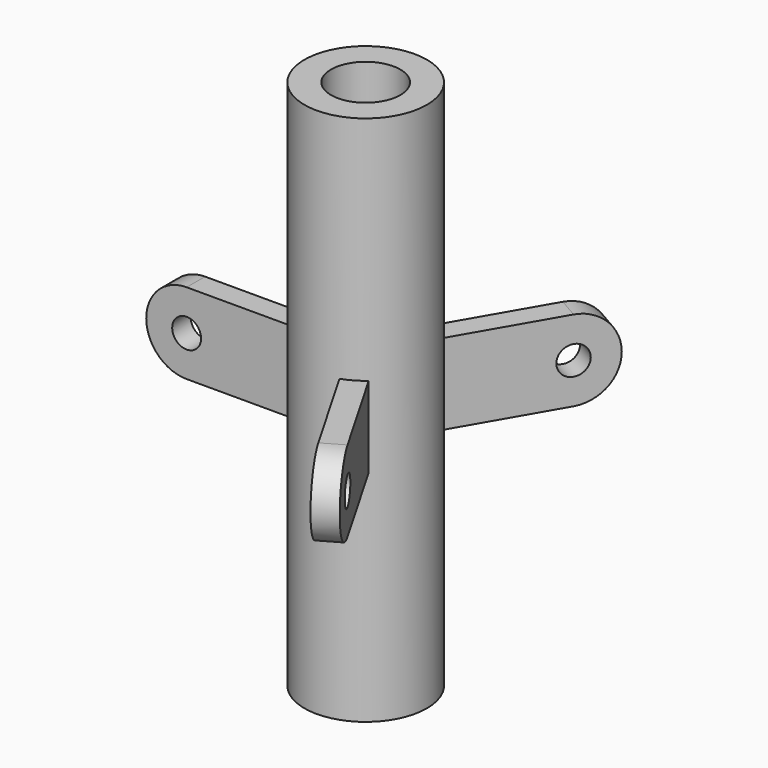
from build123d import *

# Parameters (mm, degrees)
F0_R            = 10.6
F1_DEPTH        = 92
F2_R            = 6
F3_DEPTH        = 98.1
F5_DEPTH        = 2
F5_COPIES_COUNT = 3
F7_R            = 2.5
F8_DEPTH        = 4
F9_R            = 2.5
F10_DEPTH       = 4
F11_R           = 2.5
F12_DEPTH       = 4


# Not quite as in the source:
# - a feature of the source that left no trace in its solid (it failed there, or was rolled back) is left out
# - a pattern or mirror of a feature is missing from the dataset's text; its kind, count and spacing are read off the source's solid


with BuildPart() as f1:
    # F0 (on Top) → F1 (new body)
    with BuildSketch(Plane.XY):
        Circle(F0_R)
    extrude(amount=F1_DEPTH)

    # F2 (on face) → F3 (cut)
    with BuildSketch(Plane(origin=(0, 0, 0), x_dir=(1, 0, 0), z_dir=(0, 0, -1))):
        Circle(F2_R)
    extrude(amount=-F3_DEPTH, mode=Mode.SUBTRACT)

    # F4 (on Front) → F5 (join, symmetric)
    with BuildSketch(Plane.XZ):
        with BuildLine():
            Line((-9.7803492099, 52), (-29.4, 52))
            ThreePointArc((-29.4, 52), (-36.4, 45), (-29.4, 38))
            Line((-29.4, 38), (-9.7803492099, 38))
            Line((-9.7803492099, 38), (-9.7803492099, 52))
        make_face()
    f5 = extrude(amount=F5_DEPTH, both=True)

    # F5_copies: F5 ×3 about axis
    f5_copies_axis = Axis((0, 0, 0), (0, 0, 1))
    for i in range(1, F5_COPIES_COUNT):
        add(f5.rotate(f5_copies_axis, i * 360 / F5_COPIES_COUNT))

    # F7 (on face) → F8 (cut, through all)
    with BuildSketch(Plane.XZ.offset(2)):
        with Locations((-29.4, 45)):
            Circle(F7_R)
    extrude(amount=-F8_DEPTH, mode=Mode.SUBTRACT)

    # F9 (on face) → F10 (cut, through all)
    with BuildSketch(Plane(origin=(-1.7320508076, -1, 0), x_dir=(0.5, -0.8660254038, 0), z_dir=(-0.8660254038, -0.5, 0))):
        with Locations((29.4, 45)):
            Circle(F9_R)
    extrude(amount=-F10_DEPTH, mode=Mode.SUBTRACT)

    # F11 (on face) → F12 (cut, through all)
    with BuildSketch(Plane(origin=(1.7320508076, -1, 0), x_dir=(0.5, 0.8660254038, 0), z_dir=(0.8660254038, -0.5, 0))):
        with Locations((29.4, 45)):
            Circle(F11_R)
    extrude(amount=-F12_DEPTH, mode=Mode.SUBTRACT)


solid = f1.part
